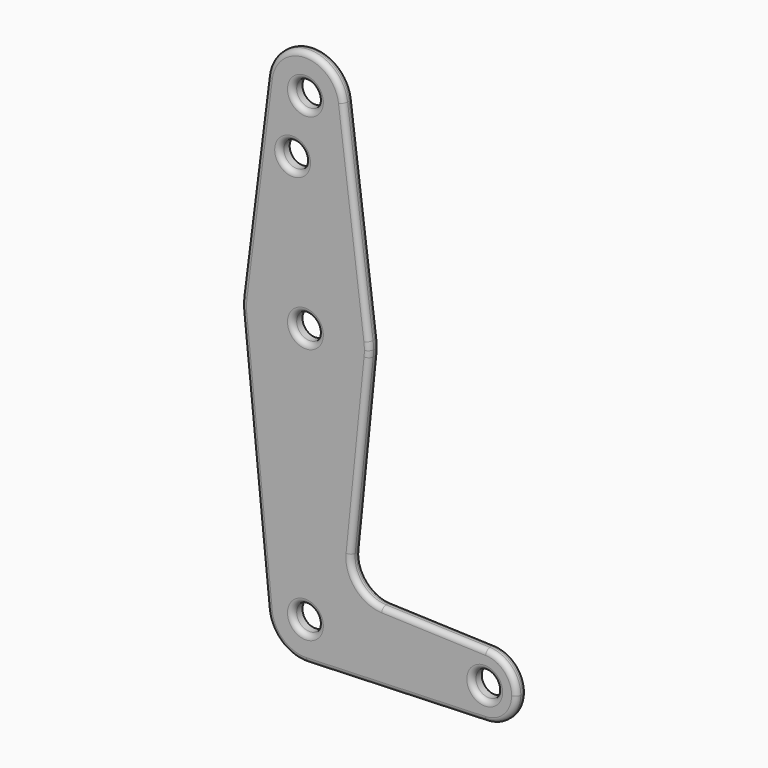
from build123d import *

# Parameters (mm, degrees)
F0_R     = 3.175
F1_DEPTH = 3.048
F2_R     = 1.27
F3_R     = 1.27


with BuildPart() as f1:
    # F0 (on Front) → F1 (new body)
    with BuildSketch(Plane.XZ):
        with BuildLine():
            ThreePointArc((44.7334821429, -7.9324362036), (50.1620069047, -5.5115227815), (52.3875, 0))
            ThreePointArc((52.3875, 0), (50.1620069047, 5.5115227815), (44.7334821429, 7.9324362036))
            ThreePointArc((44.7334821429, 7.9324362036), (36.5125, 0), (44.7334821429, -7.9324362036))
        make_face()
        with Locations((44.45, 0)):
            Circle(F0_R, mode=Mode.SUBTRACT)
        with BuildLine():
            ThreePointArc((44.7334821429, -7.9324362036), (36.5125, 0), (44.7334821429, 7.9324362036))
            Line((44.7334821429, 7.9324362036), (18.9676000005, 8.8532337108))
            ThreePointArc((18.9676000005, 8.8532337108), (13.2611998974, 11.5713591498), (11.3411865923, 17.5933818124))
            Line((11.3411865923, 17.5933818124), (15.7954255641, 61.9125))
            ThreePointArc((15.7954255641, 61.9125), (0, 47.625), (-15.7954255641, 61.9125))
            Line((-15.7954255641, 61.9125), (-9.4772553384, -0.9525))
            ThreePointArc((-9.4772553384, -0.9525), (-0.4768479324, 9.5130563464), (9.525, 0))
            ThreePointArc((9.525, 0), (6.8544082857, -6.6138273378), (0.3401785714, -9.5189234444))
            Line((0.3401785714, -9.5189234444), (44.7334821429, -7.9324362036))
        make_face()
        with BuildLine():
            ThreePointArc((-9.4772553384, -0.9525), (-6.2623833816, -7.1769199091), (0.3401785714, -9.5189234444))
            ThreePointArc((0.3401785714, -9.5189234444), (6.8544082857, -6.6138273378), (9.525, 0))
            ThreePointArc((9.525, 0), (-0.4768479324, 9.5130563464), (-9.4772553384, -0.9525))
        make_face()
        Circle(F0_R, mode=Mode.SUBTRACT)
        with BuildLine():
            ThreePointArc((-15.7954255641, 61.9125), (0, 47.625), (15.7954255641, 61.9125))
            ThreePointArc((15.7954255641, 61.9125), (15.8550939106, 62.7052534459), (15.875, 63.5))
            ThreePointArc((15.875, 63.5), (15.8438414904, 64.4941387366), (15.7504882737, 65.484375))
            ThreePointArc((15.7504882737, 65.484375), (0, 79.375), (-15.7504882737, 65.484375))
            ThreePointArc((-15.7504882737, 65.484375), (-15.8737438155, 63.6997054867), (-15.7954255641, 61.9125))
        make_face()
        with Locations((0, 63.5)):
            Circle(F0_R, mode=Mode.SUBTRACT)
        with BuildLine():
            Line((-9.4502929642, 115.490625), (-15.7504882737, 65.484375))
            ThreePointArc((-15.7504882737, 65.484375), (0, 79.375), (15.7504882737, 65.484375))
            Line((15.7504882737, 65.484375), (9.4502929642, 115.490625))
            ThreePointArc((9.4502929642, 115.490625), (9.5063048942, 114.896483242), (9.525, 114.3))
            ThreePointArc((9.525, 114.3), (-0.596483242, 104.7936951058), (-9.4502929642, 115.490625))
        make_face()
        with Locations((-3.175, 100.0252)):
            Circle(F0_R, mode=Mode.SUBTRACT)
        with BuildLine():
            ThreePointArc((9.4502929642, 115.490625), (0, 123.825), (-9.4502929642, 115.490625))
            ThreePointArc((-9.4502929642, 115.490625), (-0.596483242, 104.7936951058), (9.525, 114.3))
            ThreePointArc((9.525, 114.3), (9.5063048942, 114.896483242), (9.4502929642, 115.490625))
        make_face()
        with Locations((0, 114.3)):
            Circle(F0_R, mode=Mode.SUBTRACT)
    extrude(amount=F1_DEPTH)

    # F2
    f2_edges = [f1.edges().sort_by_distance(p)[0] for p in [
        (-12.63634, 0, 30.48),
    ]]
    fillet(f2_edges, radius=F2_R)

    # F3
    f3_edges = [f1.edges().sort_by_distance(p)[0] for p in [
        (52.3875, -3.048, 0),
        (31.850541, -3.048, 8.392835),
        (13.2612, -3.048, 11.571359),
        (13.568306, -3.048, 39.752941),
        (15.873744, -3.048, 63.699705),
        (12.600391, -3.048, 90.4875),
        (0, -3.048, 123.825),
        (-12.600391, -3.048, 90.4875),
        (-15.873744, -3.048, 63.699705),
        (-12.63634, -3.048, 30.48),
        (-6.262383, -3.048, -7.17692),
        (22.53683, -3.048, -8.72568),
        (41.275, -3.048, 0),
        (-3.175, -3.048, 0),
        (-3.175, -3.048, 63.5),
        (-6.35, -3.048, 100.0252),
        (-3.175, -3.048, 114.3),
    ]]
    fillet(f3_edges, radius=F3_R)


solid = f1.part
